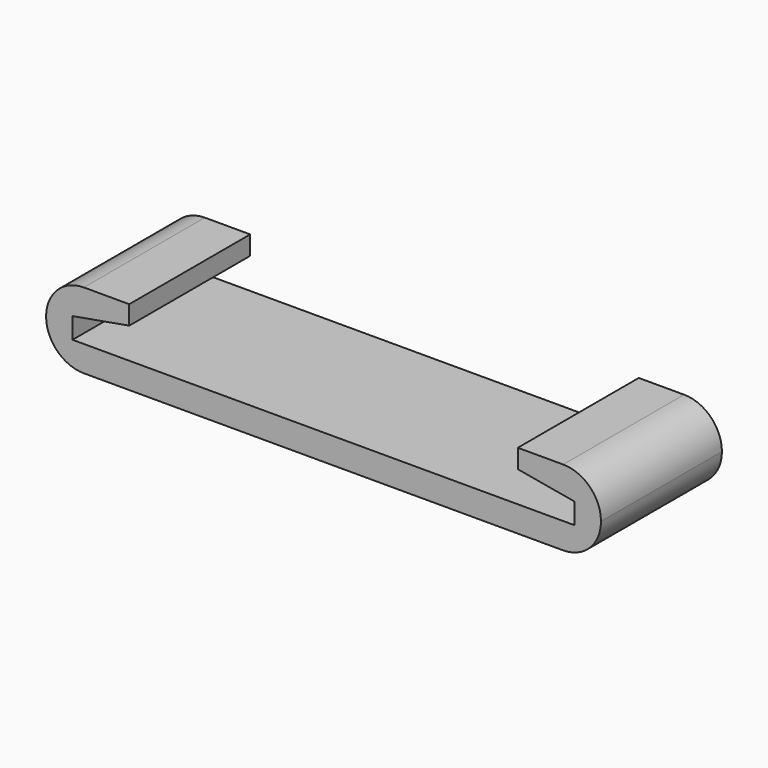
from build123d import *

# Parameters (mm, degrees)
F1_DEPTH = 25.4
F2_R     = 6.34999


# Not quite as in the source:
# - a fillet or chamfer is up to 0.001 mm smaller than in the source, because OpenCascade refuses the exact size


with BuildPart() as f1:
    # F0 (on Front) → F1 (new body)
    with BuildSketch(Plane.XZ):
        Polygon((-46.609, 0), (0, 0), (0, 4.3402855088), (-42.164, 4.3402855088), (-42.164, 7.8454855088), (-32.639, 9.525), (-32.639, 12.7), (-46.609, 12.7), align=None)
    extrude(amount=F1_DEPTH)

    # F2 (radius 6.35 in the source; OpenCascade refuses exactly that, so slightly less here)
    f2_edges = [f1.edges().sort_by_distance(p)[0] for p in [
        (-46.609, -12.7, 12.7),
        (-46.609, -12.7, 0),
    ]]
    fillet(f2_edges, radius=F2_R)

    # F3: F1 across face


with BuildPart() as f1_1:
    add(f1.part)
    add(f1.part.mirror(Plane(origin=(0, -12.7, 2.1701427544), x_dir=(0, 1, 0), z_dir=(1, 0, 0))))


solid = f1_1.part
